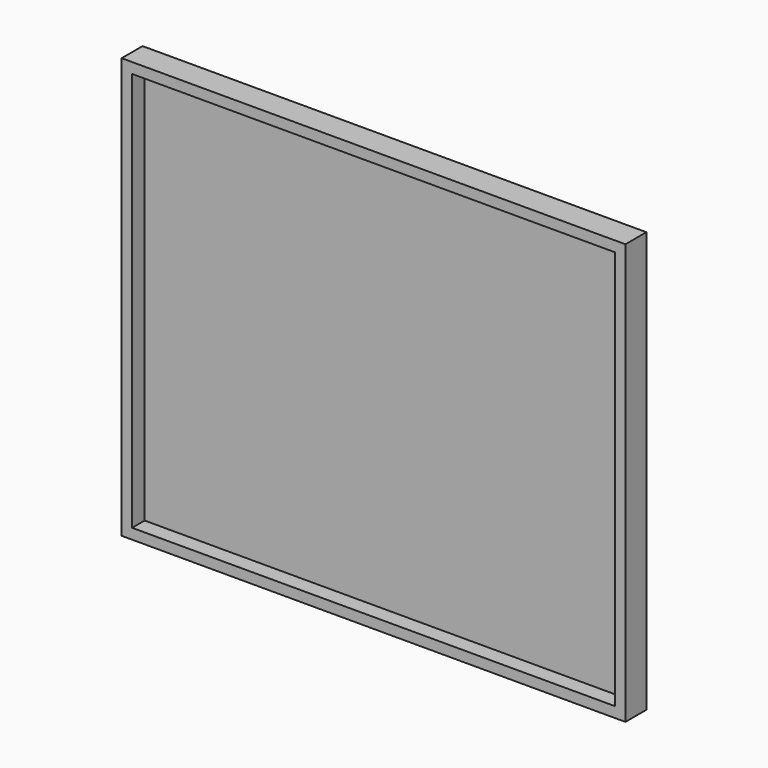
from build123d import *

# Parameters (mm, degrees)
F2_W     = 122.2148686647
F2_H     = 102.0086817443
F3_DEPTH = 6.35
F4_T     = -2.54


# Not quite as in the source:
# - the program builds the solid bodies; features that only make, move or delete a surface that nothing else refers to are left out


with BuildPart() as f3:
    # F2 (on Front) → F3 (new body)
    with BuildSketch(Plane.XZ):
        with Locations((-2.6072487235, 2.9331613332)):
            Rectangle(F2_W, F2_H)
    extrude(amount=F3_DEPTH)

    # F4
    f4_openings = [f3.faces().sort_by_distance(p)[0] for p in [
        (-2.607249, -6.35, 2.933161),
    ]]
    offset(amount=F4_T, openings=f4_openings)


solid = f3.part
